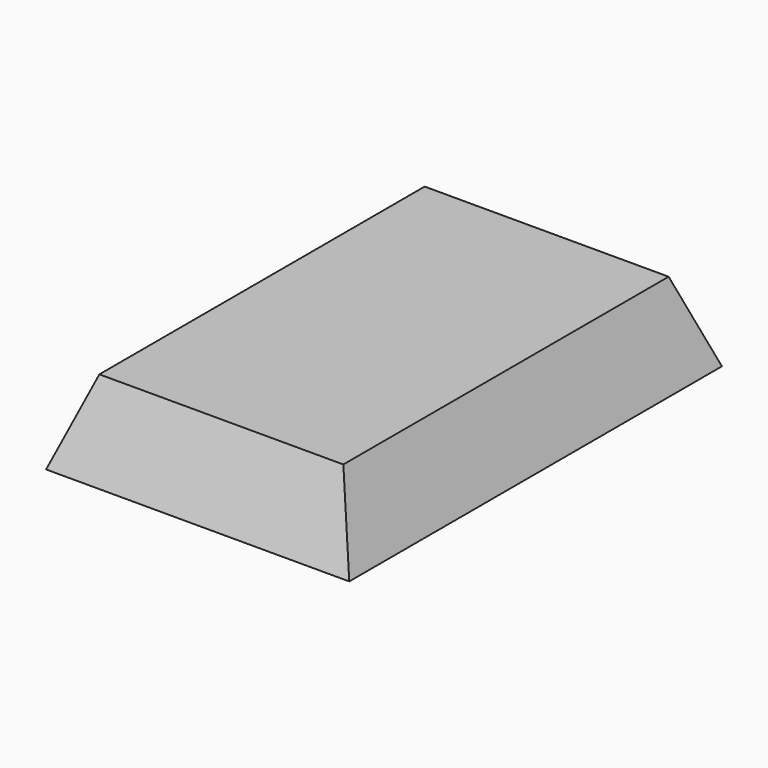
from build123d import *

# Parameters (mm, degrees)
F0_W        = 50.8
F0_H        = 76.2
F1_DEPTH    = 12.7
F2_T1_DEPTH = 166.7191414068
F2_T3_DEPTH = 141.3191414068


# Not quite as in the source:
# - a fillet or chamfer that OpenCascade refuses, or shapes differently, is made with other operations: its cross-section is extruded or revolved along the edge and cut away or added


with BuildPart() as f1:
    # F0 (on Top) → F1 (new body)
    with BuildSketch(Plane.XY):
        with Locations((25.4, 38.1)):
            Rectangle(F0_W, F0_H)
    extrude(amount=F1_DEPTH)

    # F2: chamfer of 6.35 x 17.4464816135 on 4 edges, made by hand

    # F2_s2 → F2_t1 (cut)
    with BuildSketch(Plane.XZ.offset(-121.4595707034)):
        Polygon((0, -4.7464816135), (6.35, 12.7), (0, 12.7), align=None)
        Polygon((50.8, -4.7464816135), (44.45, 12.7), (50.8, 12.7), align=None)
    extrude(amount=F2_T1_DEPTH, mode=Mode.SUBTRACT)

    # F2_s4 → F2_t3 (cut)
    with BuildSketch(Plane.YZ.offset(-45.2595707034)):
        Polygon((0, -4.7464816135), (6.35, 12.7), (0, 12.7), align=None)
        Polygon((76.2, -4.7464816135), (69.85, 12.7), (76.2, 12.7), align=None)
    extrude(amount=F2_T3_DEPTH, mode=Mode.SUBTRACT)


solid = f1.part
